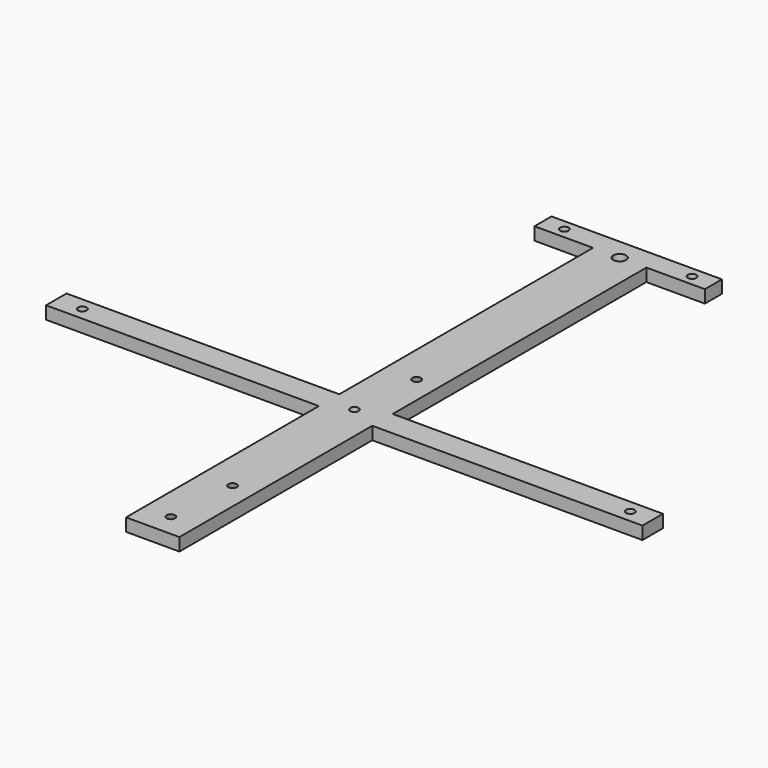
from build123d import *

# Parameters (mm, degrees)
F0_W     = 64.0446986989
F0_H     = 6
F0_R     = 1
F0_W_2   = 63.4251574627
F1_DEPTH = 3


# Not quite as in the source:
# - ends of sketch curves that miss each other by under 0.0002 mm in the source are joined
# - a feature names something its author has since deleted; it is built from what else it names


with BuildPart() as f1:
    # F0 (on Top) → F1 (new body)
    with BuildSketch(Plane.XY):
        Polygon((-7.5510093011, -42.2321148217), (-1.289947, -42.2321148217), (4.9791345373, -42.2321148217), (4.9791345373, 14.358856), (-1.595708, 14.358856), (-7.5510093011, 14.358856), align=None)
        Polygon((-0.297832, -36.78021), (-0.289947, -36.905543), (-0.297832, -37.030876), (-0.321364, -37.154233), (-0.360171, -37.273667), (-0.41364, -37.387296), (-0.48093, -37.493328), (-0.560978, -37.59009), (-0.652523, -37.676056), (-0.75412, -37.749871), (-0.864168, -37.81037), (-0.98093, -37.856599), (-1.102566, -37.88783), (-1.227157, -37.90357), (-1.352738, -37.90357), (-1.477328, -37.88783), (-1.598964, -37.856599), (-1.715726, -37.81037), (-1.825774, -37.749871), (-1.927371, -37.676056), (-2.018916, -37.59009), (-2.098964, -37.493328), (-2.166254, -37.387296), (-2.219724, -37.273667), (-2.25853, -37.154233), (-2.282062, -37.030876), (-2.289947, -36.905543), (-2.282062, -36.78021), (-2.25853, -36.656853), (-2.219724, -36.537418), (-2.166254, -36.423789), (-2.098964, -36.317758), (-2.018916, -36.220996), (-1.927371, -36.13503), (-1.825774, -36.061215), (-1.715726, -36.000716), (-1.598964, -35.954486), (-1.477328, -35.923256), (-1.352738, -35.907516), (-1.227157, -35.907516), (-1.102566, -35.923256), (-0.98093, -35.954486), (-0.864168, -36.000716), (-0.75412, -36.061215), (-0.652523, -36.13503), (-0.560978, -36.220996), (-0.48093, -36.317758), (-0.41364, -36.423789), (-0.360171, -36.537418), (-0.321364, -36.656853), align=None, mode=Mode.SUBTRACT)
        Polygon((0.834477, -20.078598), (0.842362, -20.203931), (0.834477, -20.329264), (0.810945, -20.452621), (0.772138, -20.572056), (0.718669, -20.685685), (0.651379, -20.791716), (0.571331, -20.888478), (0.479786, -20.974444), (0.378189, -21.048259), (0.268141, -21.108758), (0.151379, -21.154988), (0.029743, -21.186218), (-0.094848, -21.201958), (-0.220429, -21.201958), (-0.345019, -21.186218), (-0.466655, -21.154988), (-0.583417, -21.108758), (-0.693465, -21.048259), (-0.795062, -20.974444), (-0.886607, -20.888478), (-0.966655, -20.791716), (-1.033945, -20.685685), (-1.087415, -20.572056), (-1.126221, -20.452621), (-1.149753, -20.329264), (-1.157638, -20.203931), (-1.149753, -20.078598), (-1.126221, -19.955241), (-1.087415, -19.835807), (-1.033945, -19.722178), (-0.966655, -19.616146), (-0.886607, -19.519384), (-0.795062, -19.433418), (-0.693465, -19.359603), (-0.583417, -19.299104), (-0.466655, -19.252875), (-0.345019, -19.221644), (-0.220429, -19.205904), (-0.094848, -19.205904), (0.029743, -19.221644), (0.151379, -19.252875), (0.268141, -19.299104), (0.378189, -19.359603), (0.479786, -19.433418), (0.571331, -19.519384), (0.651379, -19.616146), (0.718669, -19.722178), (0.772138, -19.835807), (0.810945, -19.955241), align=None, mode=Mode.SUBTRACT)
        with Locations((-39.5733586505, 17.358856)):
            Rectangle(F0_W, F0_H)
        with Locations((-65.4838681221, 17.358856)):
            Circle(F0_R, mode=Mode.SUBTRACT)
        with BuildLine():
            Line((-7.5510093011, 20.358856), (-7.5510093011, 14.358856))
            Line((-7.5510093011, 14.358856), (-1.595708, 14.358856))
            Line((-1.595708, 14.358856), (-1.595708, 16.358856))
            ThreePointArc((-1.595708, 16.358856), (-2.595708, 17.358856), (-1.595708, 18.358856))
            Line((-1.595708, 18.358856), (-1.595708, 20.358856))
            Line((-1.595708, 20.358856), (-7.5510093011, 20.358856))
        make_face()
        with BuildLine():
            Line((-1.595708, 14.358856), (4.9791345373, 14.358856))
            Line((4.9791345373, 14.358856), (4.9791345373, 20.358856))
            Line((4.9791345373, 20.358856), (-1.595708, 20.358856))
            Line((-1.595708, 20.358856), (-1.595708, 18.358856))
            ThreePointArc((-1.595708, 18.358856), (-0.8886012188, 18.0659627812), (-0.595708, 17.358856))
            ThreePointArc((-0.595708, 17.358856), (-0.8886012188, 16.6517492188), (-1.595708, 16.358856))
            Line((-1.595708, 16.358856), (-1.595708, 14.358856))
        make_face()
        with Locations((36.6917132686, 17.358856)):
            Rectangle(F0_W_2, F0_H)
        with Locations((63.1569251418, 17.358856)):
            Circle(F0_R, mode=Mode.SUBTRACT)
        Polygon((-7.5510093011, 39.788339287), (-7.5510093011, 20.358856), (-1.595708, 20.358856), (4.9791345373, 20.358856), (4.9791345373, 28.8824737072), (4.9791345373, 39.788339287), (-1.289947, 39.788339287), align=None)
        Polygon((0.834477, 33.921402), (0.842362, 33.796069), (0.834477, 33.670736), (0.810945, 33.547379), (0.772138, 33.427944), (0.718669, 33.314315), (0.651379, 33.208284), (0.571331, 33.111522), (0.479786, 33.025556), (0.378189, 32.951741), (0.268141, 32.891242), (0.151379, 32.845012), (0.029743, 32.813782), (-0.094848, 32.798042), (-0.220429, 32.798042), (-0.345019, 32.813782), (-0.466655, 32.845012), (-0.583417, 32.891242), (-0.693465, 32.951741), (-0.795062, 33.025556), (-0.886607, 33.111522), (-0.966655, 33.208284), (-1.033945, 33.314315), (-1.087415, 33.427944), (-1.126221, 33.547379), (-1.149753, 33.670736), (-1.157638, 33.796069), (-1.149753, 33.921402), (-1.126221, 34.044759), (-1.087415, 34.164193), (-1.033945, 34.277822), (-0.966655, 34.383854), (-0.886607, 34.480616), (-0.795062, 34.566582), (-0.693465, 34.640397), (-0.583417, 34.700896), (-0.466655, 34.747125), (-0.345019, 34.778356), (-0.220429, 34.794096), (-0.094848, 34.794096), (0.029743, 34.778356), (0.151379, 34.747125), (0.268141, 34.700896), (0.378189, 34.640397), (0.479786, 34.566582), (0.571331, 34.480616), (0.651379, 34.383854), (0.718669, 34.277822), (0.772138, 34.164193), (0.810945, 34.044759), align=None, mode=Mode.SUBTRACT)
        with BuildLine():
            Line((-7.5510093011, 94.7883501649), (-7.5510093011, 39.788339287))
            Line((-7.5510093011, 39.788339287), (-1.289947, 39.788339287))
            Line((-1.289947, 39.788339287), (4.9791345373, 39.788339287))
            Line((4.9791345373, 39.788339287), (4.9791345373, 94.7883501649))
            Line((4.9791345373, 94.7883501649), (0.2140626181, 94.7883501649))
            ThreePointArc((0.2140626181, 94.7883501649), (-1.2859428208, 93.2883392871), (-2.7859373819, 94.7883501649))
            Line((-2.7859373819, 94.7883501649), (-7.5510093011, 94.7883501649))
        make_face()
        Polygon((-21.2859819876, 94.7883501649), (-7.5510093011, 94.7883501649), (-7.5510093011, 99.788339287), (-21.2859819876, 99.7883501649), align=None)
        with Locations((-16.2859819876, 97.2883501649)):
            Circle(F0_R, mode=Mode.SUBTRACT)
        with BuildLine():
            Line((-7.5510093011, 99.788339287), (-7.5510093011, 94.7883501649))
            Line((-7.5510093011, 94.7883501649), (-2.7859373819, 94.7883501649))
            ThreePointArc((-2.7859373819, 94.7883501649), (-1.285931943, 96.288339287), (0.2140626181, 94.788339287))
            Line((0.2140626181, 94.788339287), (4.9791345373, 94.7883501649))
            Line((4.9791345373, 94.7883501649), (4.9791345373, 99.788339287))
            Line((4.9791345373, 99.788339287), (-7.5510093011, 99.788339287))
        make_face()
        Polygon((4.9791345373, 99.788339287), (4.9791345373, 94.7883501649), (18.7140180124, 94.7883501649), (18.7140180124, 99.7883501649), align=None)
        with Locations((13.7140180124, 97.2883501649)):
            Circle(F0_R, mode=Mode.SUBTRACT)
    extrude(amount=F1_DEPTH)


solid = f1.part
